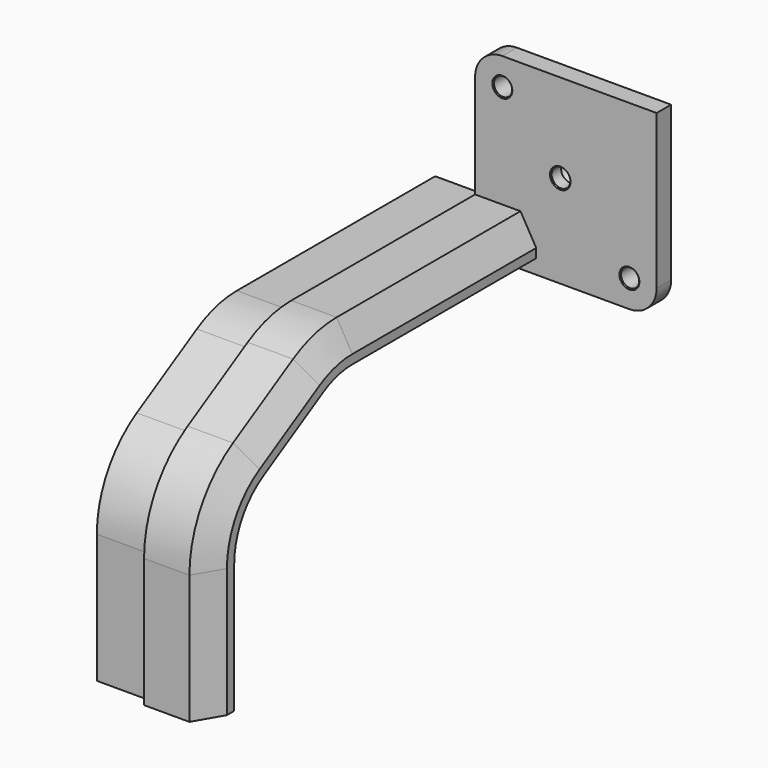
from build123d import *

# Parameters (mm, degrees)
F0_R     = 5
F1_DEPTH = 10
F3_D     = 10.3
F3_DEPTH = 7
F3_TIP   = 3.094432188
F4_SIZE  = 0.5


with BuildPart() as f1:
    # F0 (on Front) → F1 (new body)
    with BuildSketch(Plane.XZ):
        with BuildLine():
            Line((0, 85), (0, 0))
            Line((0, 0), (85, 0))
            ThreePointArc((85, 0), (95.6066017178, 4.3933982822), (100, 15))
            Line((100, 15), (100, 100))
            Line((100, 100), (15, 100))
            ThreePointArc((15, 100), (4.3933982822, 95.6066017178), (0, 85))
        make_face()
        with Locations((85, 15)):
            Circle(F0_R, mode=Mode.SUBTRACT)
        with Locations((15, 85)):
            Circle(F0_R, mode=Mode.SUBTRACT)
    extrude(amount=F1_DEPTH)

    # F3
    with Locations(Plane.XZ.offset(10)):
        with Locations((46.9228513539, 51.1608496308)):
            Hole(F3_D / 2, depth=F3_DEPTH)
            with Locations((0, 0, -(F3_DEPTH + F3_TIP / 2))):  # 118° drill point
                Cone(0, F3_D / 2, F3_TIP, mode=Mode.SUBTRACT)

    # F4
    f4_edges = [f1.edges().sort_by_distance(p)[0] for p in [
        (10, -10, 85),
        (80, -10, 15),
        (41.772851, -10, 51.16085),
    ]]
    chamfer(f4_edges, length=F4_SIZE)


with BuildPart() as f7:
    # F7: sweep along a path in F6
    with BuildLine(Plane.YZ) as f7_path:
        Line((0, 18), (-136.6025403784, 18))
        ThreePointArc((-136.6025403784, 18), (-149.5434926336, 16.2962913145), (-161.6025403784, 11.3012701892))
        Line((-161.6025403784, 11.3012701892), (-202.9422863406, -12.5662432703))
        ThreePointArc((-202.9422863406, -12.5662432703), (-221.2435565298, -30.8675134595), (-227.9422863406, -55.8675134595))
        Line((-227.9422863406, -55.8675134595), (-227.9422863406, -127))
    # F5 (on Front) → F7 (sweep)
    with BuildSketch(Plane.XZ):
        Polygon((-30, 23), (-30, 18), (20, 18), (20, 8), (33.6602540378, 8), (33.6602540378, 13), (25, 28), (0, 28), (0, 23), align=None)
    sweep(path=f7_path.line)


solid = Compound([f1.part, f7.part])
